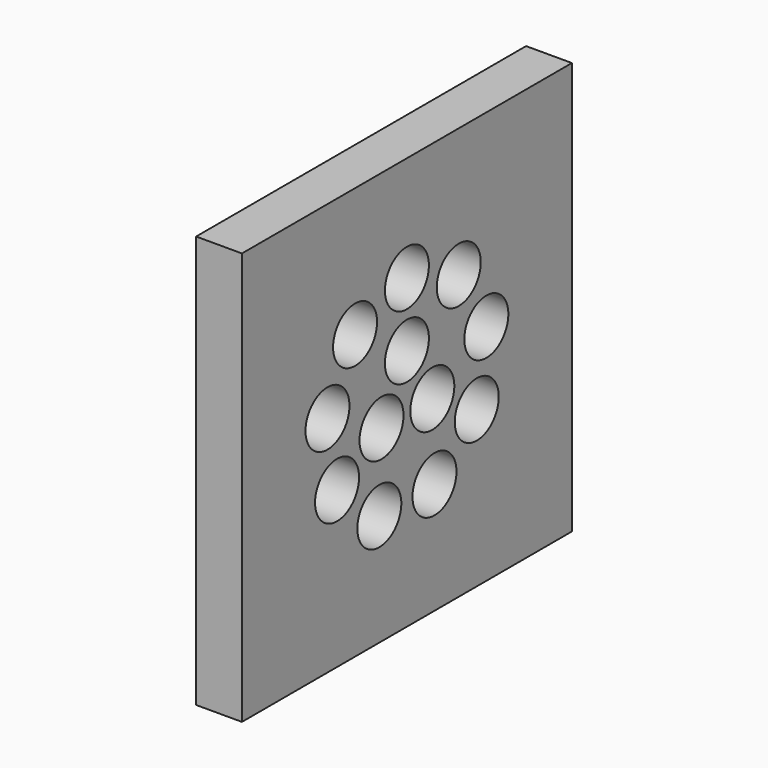
from build123d import *

# Parameters (mm, degrees)
F2_W     = 90
F2_H     = 90
F3_DEPTH = 10
F4_D     = 12
F4_DEPTH = 20
F4_TIP   = 3.6051637142


# Not quite as in the source:
# - a feature names something its author has since deleted; it is built from what else it names


with BuildPart() as f1:
    # F0 (on Front) → F1 (revolve)
    with BuildSketch(Plane.XZ):
        Polygon((-14.3225658685, 0), (-10, 0), (-10, 32.5), (-10, 39), (-14.3225658685, 39), (-14.3225658685, 34.4556160271), (-14.3225658685, 32.5), align=None)
    revolve(axis=Axis((-45.5725640059, 0, 0), (-1, 0, 0)))

    # F2 (on Right) → F3 (join)
    with BuildSketch(Plane.YZ):
        Rectangle(F2_W, F2_H)
    extrude(amount=-F3_DEPTH)

    # F4
    with Locations(Plane.YZ):
        with Locations((-6.9282032303, -4), (6.9282032303, -4), (0, 8), (-21.6657705663, 3.8202599087), (-14.1413274131, 16.8529777486), (0, 22), (14.1413274131, 16.8529777486), (21.6657705663, 3.8202599087), (19.0525588833, -11), (7.5244431532, -20.6732376573), (-7.5244431532, -20.6732376573), (-19.0525588833, -11)):
            Hole(F4_D / 2, depth=F4_DEPTH)
            with Locations((0, 0, -(F4_DEPTH + F4_TIP / 2))):  # 118° drill point
                Cone(0, F4_D / 2, F4_TIP, mode=Mode.SUBTRACT)


solid = f1.part
